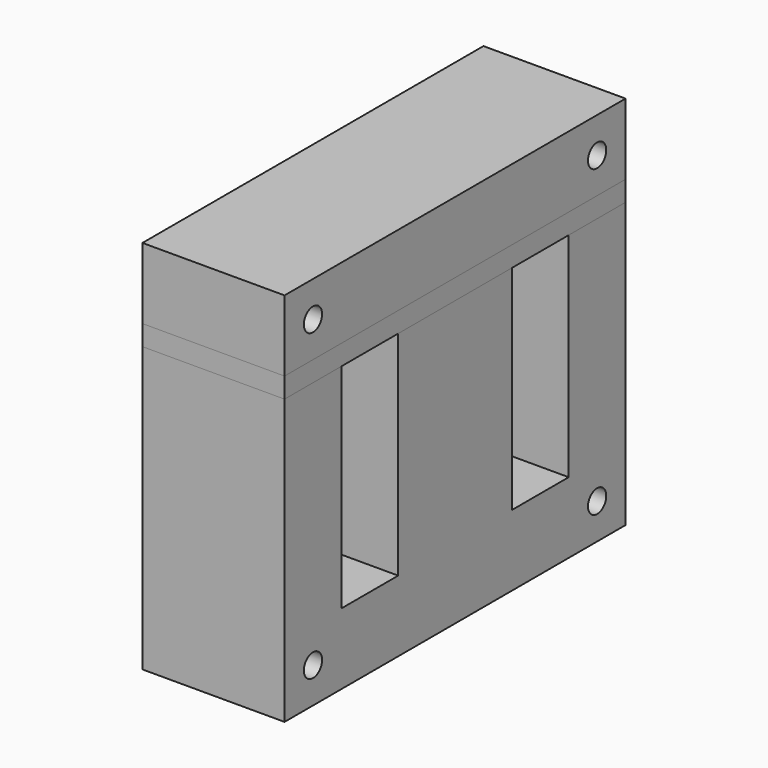
from build123d import *

# Parameters (mm, degrees)
F2_W      = 44.45
F2_H      = 133.35
F3_DEPTH  = 88.9
F4_W      = 44.45
F4_H      = 22.225
F5_DEPTH  = 66.675
F6_R      = 3.571875
F7_DEPTH  = 44.45
F8_W      = 44.45
F8_H      = 133.35
F9_DEPTH  = 6.35
F10_W     = 44.45
F10_H     = 133.35
F11_DEPTH = 22.225
F12_R     = 3.571875
F13_DEPTH = 44.45


# Not quite as in the source:
# - a variable given as a bare number and used for a length is read in inches; the dataset says mm whatever the document's units were


with BuildPart() as f3:
    # F2 (on Top) → F3 (new body)
    with BuildSketch(Plane.XY):
        Rectangle(F2_W, F2_H)
    extrude(amount=F3_DEPTH)

    # F4 (on face) → F5 (cut)
    with BuildSketch(Plane.XY.offset(88.9)):
        with Locations((0, -33.3375)):
            Rectangle(F4_W, F4_H)
        with Locations((0, 33.3375)):
            Rectangle(F4_W, F4_H)
    extrude(amount=-F5_DEPTH, mode=Mode.SUBTRACT)

    # F6 (on face) → F7 (cut)
    with BuildSketch(Plane(origin=(-22.225, 0, 0), x_dir=(0, -1, 0), z_dir=(-1, 0, 0))):
        with Locations((-55.5625, 11.1125)):
            Circle(F6_R)
        with Locations((55.5625, 11.1125)):
            Circle(F6_R)
    extrude(amount=-F7_DEPTH, mode=Mode.SUBTRACT)


with BuildPart() as f9:
    # F8 (on face) → F9 (new body)
    with BuildSketch(Plane.XY.offset(88.9)):
        Rectangle(F8_W, F8_H)
    extrude(amount=F9_DEPTH)


with BuildPart() as f11:
    # F10 (on face) → F11 (new body)
    with BuildSketch(Plane.XY.offset(95.25)):
        Rectangle(F10_W, F10_H)
    extrude(amount=F11_DEPTH)

    # F12 (on face) → F13 (cut)
    with BuildSketch(Plane(origin=(-22.225, 0, 0), x_dir=(0, -1, 0), z_dir=(-1, 0, 0))):
        with Locations((-55.5625, 106.3625)):
            Circle(F12_R)
        with Locations((55.5625, 106.3625)):
            Circle(F12_R)
    extrude(amount=-F13_DEPTH, mode=Mode.SUBTRACT)


solid = Compound([f3.part, f9.part, f11.part])
